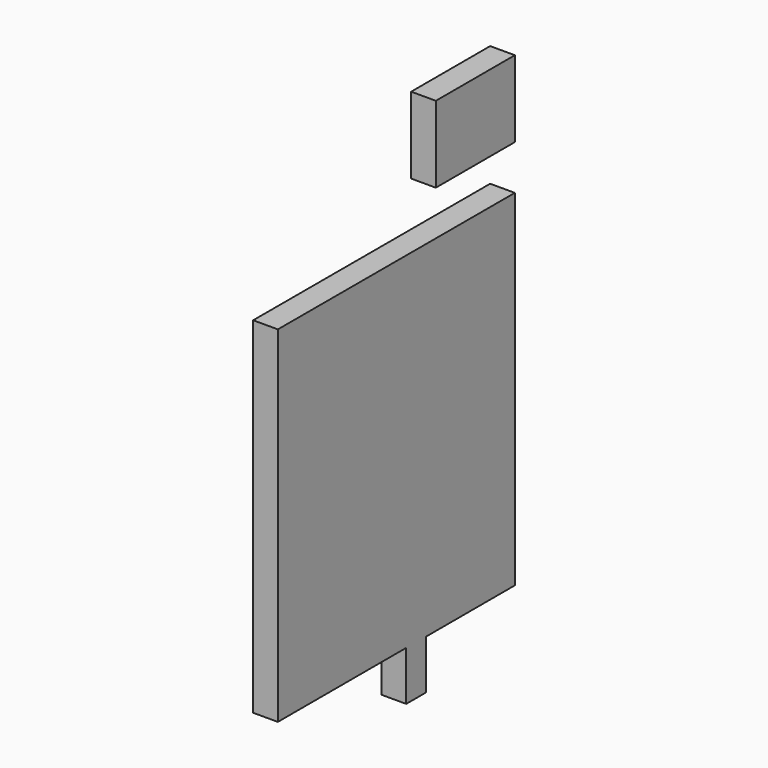
from build123d import *

# Parameters (mm, degrees)
F1_DEPTH = 5


# Not quite as in the source:
# - a feature names something its author has since deleted; it is built from what else it names


with BuildPart() as f1:
    # F0 (on Right) → F1 (new body)
    with BuildSketch(Plane.YZ):
        Polygon((60, -0.0434386059), (0, 0), (0, -70), (12, -70), (12.4011761725, -70), (32.5, -70), (32.5, -80), (37.5, -80), (37.5, -70.0434386059), (60, -70.0434386059), align=None)
    extrude(amount=F1_DEPTH)


with BuildPart() as f1b:
    # F0 (on Right) → F1, piece 2 (new body)
    with BuildSketch(Plane.YZ):
        Polygon((40, 8.9999613941), (42.5, 8.9999613941), (60, 8.9999613941), (60, 24.499980697), (42.5, 24.499980697), (40, 24.499980697), align=None)
    extrude(amount=F1_DEPTH)


solid = Compound([f1.part, f1b.part])
